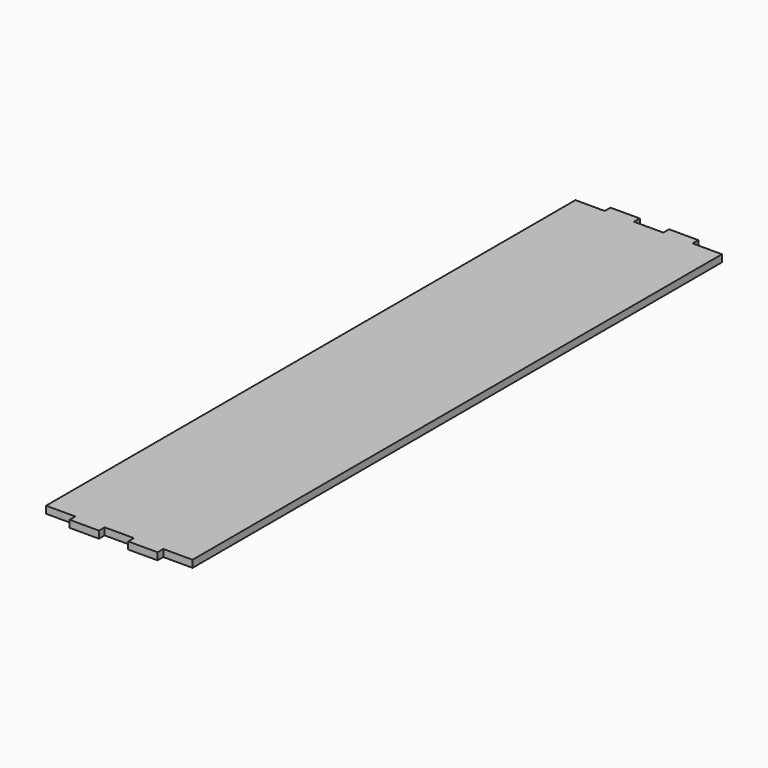
from build123d import *

# Parameters (mm, degrees)
F0_W     = 65
F0_H     = 300
F1_DEPTH = 3.175
F2_W     = 13
F2_H     = 3.175
F3_DEPTH = 3.176


# Not quite as in the source:
# - a length typed as a fraction of an inch, garbled in the dataset ("3 / 203.2 mm" for 3/8 in), is restored


with BuildPart() as f1:
    # F0 (on Top) → F1 (new body)
    with BuildSketch(Plane.XY):
        Rectangle(F0_W, F0_H)
    extrude(amount=F1_DEPTH)

    # F2 (on face) → F3 (cut, through all)
    with BuildSketch(Plane.XY.offset(3.175)):
        with Locations((-26, -148.4125)):
            Rectangle(F2_W, F2_H)
        with Locations((-26, 148.4125)):
            Rectangle(F2_W, F2_H)
        with Locations((0, -148.4125)):
            Rectangle(F2_W, F2_H)
        with Locations((0, 148.4125)):
            Rectangle(F2_W, F2_H)
        with Locations((26, -148.4125)):
            Rectangle(F2_W, F2_H)
        with Locations((26, 148.4125)):
            Rectangle(F2_W, F2_H)
    extrude(amount=-F3_DEPTH, mode=Mode.SUBTRACT)


solid = f1.part
